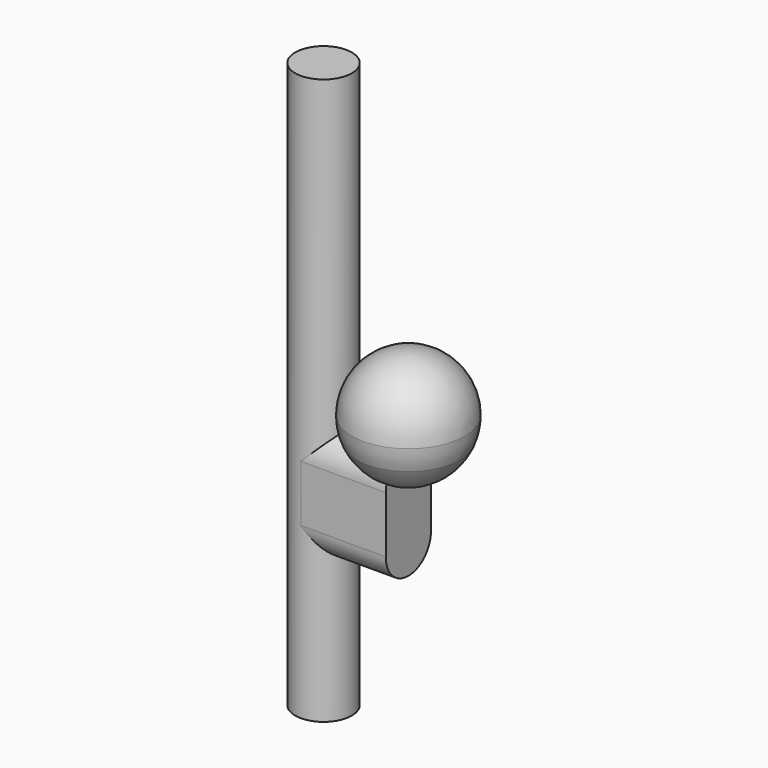
from build123d import *

# Parameters (mm, degrees)
F0_R     = 12.7
F2_DEPTH = 127
F4_DEPTH = 38.1


# Not quite as in the source:
# - the program builds the solid bodies; features that only make, move or delete a surface that nothing else refers to are left out


with BuildPart() as f2:
    # F0 (on Top) → F2 (new body, symmetric)
    with BuildSketch(Plane.XY):
        with Locations((-38.1, 0)):
            Circle(F0_R)
    extrude(amount=F2_DEPTH, both=True)


with BuildPart() as f4:
    # F3 (on Right) → F4 (new body)
    with BuildSketch(Plane.YZ):
        with BuildLine():
            ThreePointArc((-12.7, -25.4), (0, -38.1), (12.7, -25.4))
            ThreePointArc((12.7, -25.4), (0, -12.7), (-12.7, -25.4))
        make_face()
        with BuildLine():
            Line((12.7, -50.8), (12.7, -25.4))
            ThreePointArc((12.7, -25.4), (0, -38.1), (-12.7, -25.4))
            Line((-12.7, -25.4), (-12.7, -50.8))
            Line((-12.7, -50.8), (12.7, -50.8))
        make_face()
        with BuildLine():
            ThreePointArc((-12.7, -50.8), (0, -63.5), (12.7, -50.8))
            Line((12.7, -50.8), (-12.7, -50.8))
        make_face()
    extrude(amount=-F4_DEPTH)


with BuildPart() as f8:
    # F7 (on Front) → F8 (revolve)
    with BuildSketch(Plane.XZ):
        with BuildLine():
            ThreePointArc((23.2794845304, -10.16), (24.8642203484, -5.1894649497), (25.4, 0))
            ThreePointArc((25.4, 0), (17.9605122421, 17.9605122421), (0, 25.4))
            Line((0, 25.4), (0, -10.16))
            Line((0, -10.16), (23.2794845304, -10.16))
        make_face()
        with BuildLine():
            ThreePointArc((0, -25.4), (13.9121529606, -21.251164674), (23.2794845304, -10.16))
            Line((23.2794845304, -10.16), (0, -10.16))
            Line((0, -10.16), (0, -25.4))
        make_face()
    revolve(axis=Axis((0, 0, 0), (0, 0, 1)))


solid = Compound([f2.part, f4.part, f8.part])
